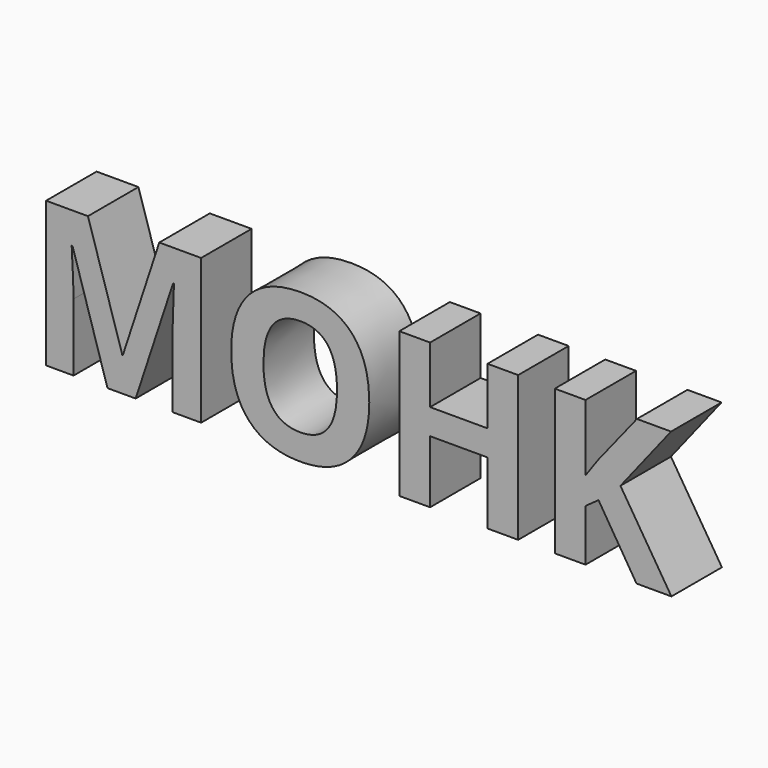
from build123d import *

# Parameters (mm, degrees)
F0_TEXT_SIZE = 81.7655747394
F1_DEPTH     = 25.4


# Not quite as in the source:
# - Text() gives the source's letters only with a copy of the font that has no kerning and outlines rounded to 1/6400 em; it was checked with that copy


with BuildPart() as f1:
    # F0 (on Front) → F1 (new body)
    with BuildSketch(Plane.XZ):
        with Locations((-199.6455341578, -6.9922064431)):
            Text('MOHK', F0_TEXT_SIZE, font='Open Sans', font_style=FontStyle.BOLD, text_align=(TextAlign.LEFT, TextAlign.BOTTOM))
    extrude(amount=F1_DEPTH)


solid = f1.part
